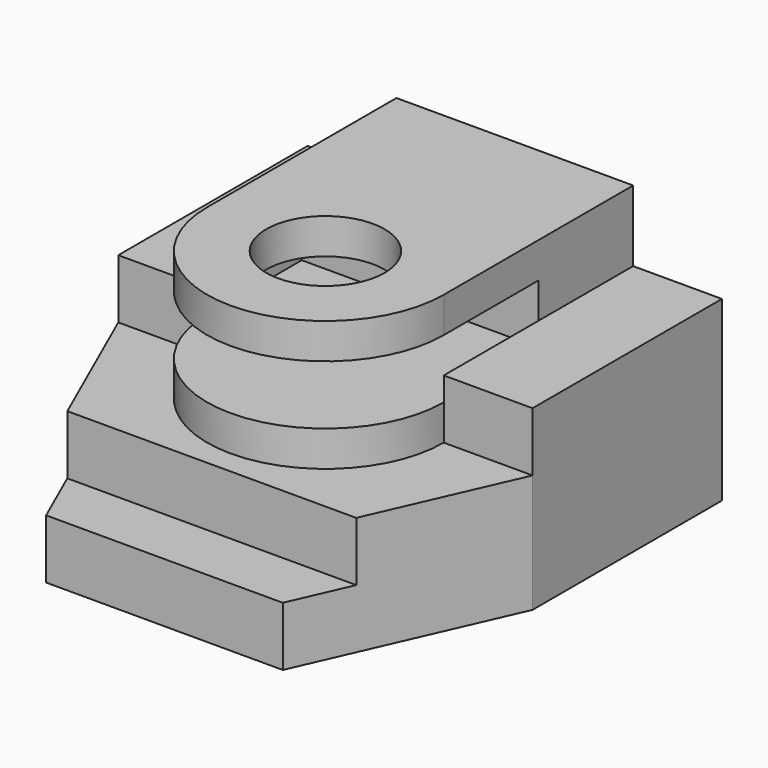
from build123d import *

# Parameters (mm, degrees)
F1_DEPTH       = 22
F3_R           = 10
F4_DEPTH       = 6
F6_DEPTH       = 20
F7_W           = 10
F7_H           = 10
F8_DEPTH       = 55.001
F8_DEPTH_BACK  = 15.001
F9_W           = 40
F9_H           = 30
F10_DEPTH      = 15
F10_DEPTH_BACK = 55
F2_W           = 40
F2_H           = 10
F11_DEPTH      = 40


# Not quite as in the source:
# - an extrude ends at something that could not be found from the text; its depth is read off the source's solid


with BuildPart() as f1:
    # F0 (on Top) → F1 (new body)
    with BuildSketch(Plane.XY):
        with BuildLine():
            Line((40, 18.5987265639), (0, 18.5987265639))
            Line((0, 18.5987265639), (0, -21.4012734361))
            ThreePointArc((0, -21.4012734361), (20, -41.4012734361), (40, -21.4012734361))
            Line((40, -21.4012734361), (40, 18.5987265639))
        make_face()
    extrude(amount=F1_DEPTH)

    # F3 (on face) → F4 (cut)
    with BuildSketch(Plane.XY.offset(22)):
        with Locations((20, -21.4012734361)):
            Circle(F3_R)
    extrude(amount=-F4_DEPTH, mode=Mode.SUBTRACT)

    # F5 (on face) → F6 (join)
    with BuildSketch(Plane(origin=(0, 0, 0), x_dir=(1, 0, 0), z_dir=(0, 0, -1))):
        Polygon((0, 55.4012734361), (-15, 21.4012734361), (55, 21.4012734361), (40, 55.4012734361), align=None)
    extrude(amount=F6_DEPTH)

    # F7 (on face) → F8 (cut, two sides)
    with BuildSketch(Plane.YZ.offset(40)) as f8_sk:
        with Locations((-50.4012734361, -5)):
            Rectangle(F7_W, F7_H)
    extrude(amount=-F8_DEPTH, mode=Mode.SUBTRACT)
    extrude(f8_sk.sketch, amount=F8_DEPTH_BACK, mode=Mode.SUBTRACT)

    # F9 (on face) → F10 (join, two sides)
    with BuildSketch(Plane.YZ.offset(40)) as f10_sk:
        with Locations((-1.4012734361, -5)):
            Rectangle(F9_W, F9_H)
    extrude(amount=F10_DEPTH)
    extrude(f10_sk.sketch, amount=-F10_DEPTH_BACK)

    # F2 (on face) → F11 (cut, through all)
    with BuildSketch(Plane.YZ.offset(40)):
        with Locations((-21.4012734361, 11)):
            Rectangle(F2_W, F2_H)
    extrude(amount=-F11_DEPTH, mode=Mode.SUBTRACT)


solid = f1.part
